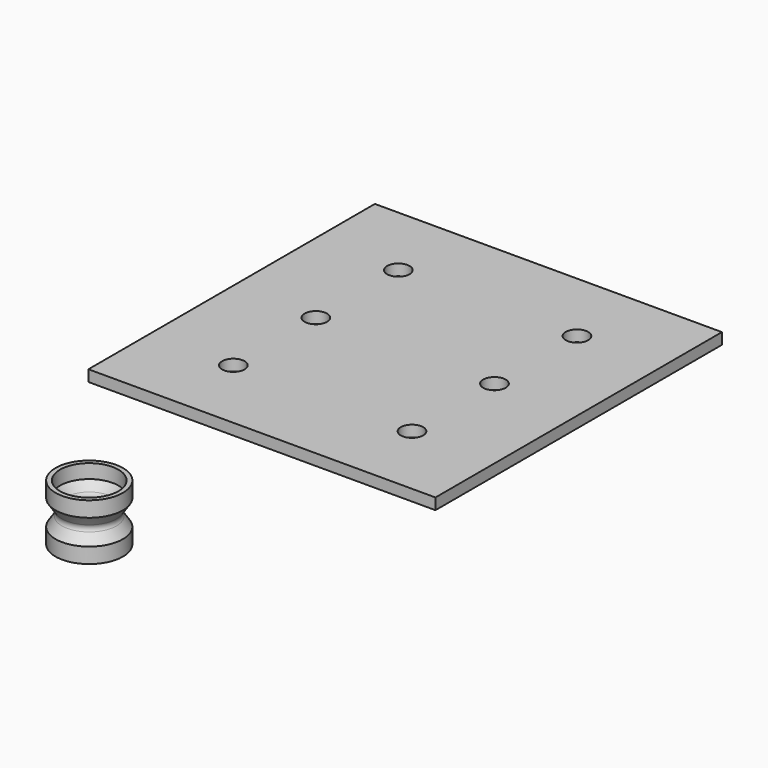
from build123d import *

# Parameters (mm, degrees)
F0_W     = 61.8
F0_H     = 100.8965958967
F1_DEPTH = 5
F4_R     = 2
F4_W     = 61.8
F4_H     = 18.5648719378
F5_DEPTH = 25
F7_DEPTH = 3


with BuildPart() as f1:
    # F0 (on Top) → F1 (new body)
    with BuildSketch(Plane.XY):
        Rectangle(F0_W, F0_H)
    extrude(amount=F1_DEPTH)

    # F4 (on face) → F5 (cut)
    with BuildSketch(Plane.XY.offset(5)):
        with Locations((-15.9011339205, 0)):
            Circle(F4_R)
        with Locations((-15.9011339205, -18.3610478988)):
            Circle(F4_R)
        with Locations((15.9011339205, 18.3610478988)):
            Circle(F4_R)
        with Locations((15.9011339205, 0)):
            Circle(F4_R)
        with Locations((15.9011339205, -18.3610478988)):
            Circle(F4_R)
        with Locations((-15.9011339205, 18.3610478988)):
            Circle(F4_R)
        with Locations((0, 41.1658619795)):
            Rectangle(F4_W, F4_H)
        with Locations((0, -41.1658619795)):
            Rectangle(F4_W, F4_H)
    extrude(amount=-F5_DEPTH, mode=Mode.SUBTRACT)

    # F7 (cut): a face of the model
    f7_faces = [f1.faces().sort_by_distance(p)[0] for p in [
        (0, 0, 0),
    ]]
    extrude(f7_faces, amount=-F7_DEPTH, mode=Mode.SUBTRACT)


with BuildPart() as f3:
    # F2 (on face) → F3 (revolve)
    with BuildSketch(Plane.XZ.offset(50.4482979484)):
        with BuildLine():
            Line((-9.9011339205, 0), (-10.7011339205, 0))
            Line((-10.7011339205, 0), (-10.7011339205, -2.5))
            Line((-10.7011339205, -2.5), (-11.7001136063, -4.0041586889))
            ThreePointArc((-11.7001136063, -4.0041586889), (-12.0006803523, -5), (-11.7001136063, -5.9958413111))
            Line((-11.7001136063, -5.9958413111), (-10.7011339205, -7.5))
            Line((-10.7011339205, -7.5), (-10.7011339205, -10))
            Line((-10.7011339205, -10), (-9.9011339205, -10))
            Line((-9.9011339205, -10), (-9.9011339205, -7.2585424564))
            Line((-9.9011339205, -7.2585424564), (-11.0336988267, -5.5532451728))
            ThreePointArc((-11.0336988267, -5.5532451728), (-11.2006803523, -5), (-11.0336988267, -4.4467548272))
            Line((-11.0336988267, -4.4467548272), (-9.9011339205, -2.7414575436))
            Line((-9.9011339205, -2.7414575436), (-9.9011339205, 0))
        make_face()
    revolve(axis=Axis((-15.9011339205, -50.4482979484, -5), (0, 0, -1)))


solid = Compound([f1.part, f3.part])
